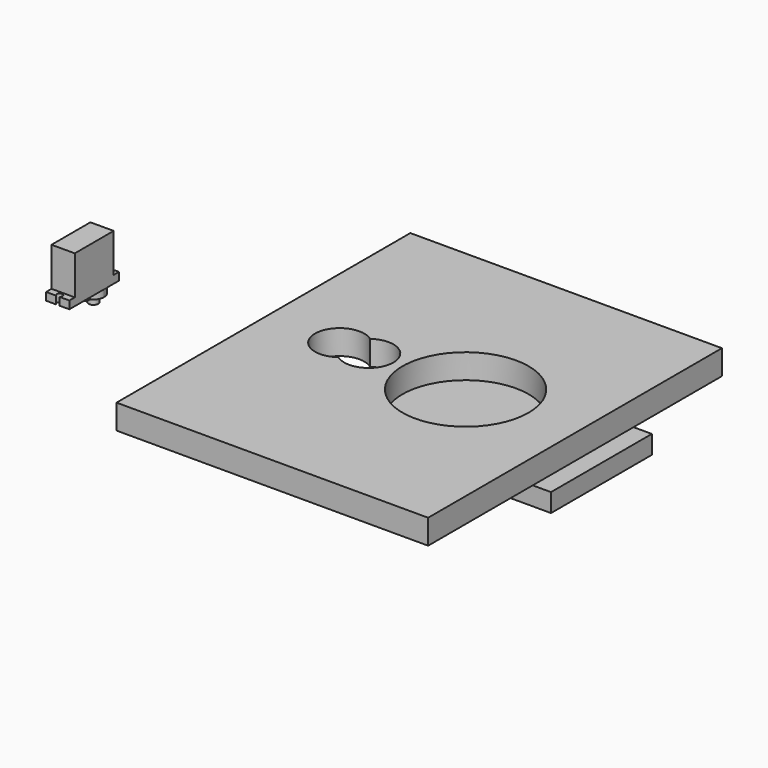
from build123d import *

# Parameters (mm, degrees)
F0_W      = 160.6854679329
F0_H      = 189.3717367202
F0_R      = 32.5
F1_DEPTH  = 12.7
F2_W      = 124
F2_H      = 65
F3_DEPTH  = 9.525
F5_DEPTH  = 12.7
F6_R      = 2.5
F7_DEPTH  = 24
F8_DEPTH  = 4
F9_DEPTH  = 8
F11_DEPTH = 20
F12_DEPTH = 4


# Not quite as in the source:
# - a length typed as a fraction of an inch, garbled in the dataset ("3 / 203.2 mm" for 3/8 in), is restored


with BuildPart() as f1:
    # F0 (on Top) → F1 (new body)
    with BuildSketch(Plane.XY):
        with Locations((-1.9587278366, 0.8332561702)):
            Rectangle(F0_W, F0_H)
        with Locations((20.2750398644, 2.9224749887)):
            Circle(F0_R, mode=Mode.SUBTRACT)
    extrude(amount=F1_DEPTH)

    # F4 (on face) → F5 (cut, through all)
    with BuildSketch(Plane.XY.offset(12.7)):
        with BuildLine():
            ThreePointArc((-37.3042601347, -7.1310623929), (-24.0579569753, -8.2077946527), (-17.1042601347, 3.1178399874))
            ThreePointArc((-17.1042601347, 3.1178399874), (-24.0579569753, 14.4434746274), (-37.3042601347, 13.3667423676))
            ThreePointArc((-37.3042601347, 13.3667423676), (-33.4786254946, 8.8641431468), (-32.1042601347, 3.1178399874))
            ThreePointArc((-32.1042601347, 3.1178399874), (-33.4786254946, -2.628463172), (-37.3042601347, -7.1310623929))
        make_face()
        with BuildLine():
            ThreePointArc((-32.1042601347, 3.1178399874), (-33.4786254946, 8.8641431468), (-37.3042601347, 13.3667423676))
            ThreePointArc((-37.3042601347, 13.3667423676), (-42.5042601347, 3.1178399874), (-37.3042601347, -7.1310623929))
            ThreePointArc((-37.3042601347, -7.1310623929), (-33.4786254946, -2.628463172), (-32.1042601347, 3.1178399874))
        make_face()
        with BuildLine():
            ThreePointArc((-37.3042601347, -7.1310623929), (-42.5042601347, 3.1178399874), (-37.3042601347, 13.3667423676))
            ThreePointArc((-37.3042601347, 13.3667423676), (-57.5042601347, 3.1178399874), (-37.3042601347, -7.1310623929))
        make_face()
    extrude(amount=-F5_DEPTH, mode=Mode.SUBTRACT)


with BuildPart() as f3:
    # F2 (on Top) → F3 (new body)
    with BuildSketch(Plane.XY):
        with Locations((25.8148865969, 6.0524680488)):
            Rectangle(F2_W, F2_H)
    extrude(amount=-F3_DEPTH)


with BuildPart() as f7:
    # F6 (on Top) → F7 (new body)
    with BuildSketch(Plane.XY):
        with BuildLine():
            Line((-170.091433923, 8.8584844804), (-175.1961884499, 8.8584844804))
            Line((-175.1961884499, 8.8584844804), (-175.1961884499, -23.1415155196))
            Line((-175.1961884499, -23.1415155196), (-170.091433923, -23.1415155196))
            ThreePointArc((-170.091433923, -23.1415155196), (-169.8696614598, -20.5976531011), (-167.6961884499, -21.9379642981))
            ThreePointArc((-167.6961884499, -21.9379642981), (-167.8558772528, -22.611437308), (-168.3009429767, -23.1415155196))
            Line((-168.3009429767, -23.1415155196), (-163.1961884499, -23.1415155196))
            Line((-163.1961884499, -23.1415155196), (-163.1961884499, 8.8584844804))
            Line((-163.1961884499, 8.8584844804), (-168.3009429767, 8.8584844804))
            ThreePointArc((-168.3009429767, 8.8584844804), (-167.8558772528, 8.3284062688), (-167.6961884499, 7.6549332589))
            ThreePointArc((-167.6961884499, 7.6549332589), (-169.8696614598, 6.3146220619), (-170.091433923, 8.8584844804))
        make_face()
        with BuildLine():
            ThreePointArc((-172.1793124567, -4.7622266293), (-171.827045531, 4.6884524947), (-163.6961884499, -0.1415155196))
            ThreePointArc((-163.6961884499, -0.1415155196), (-164.5558902937, -3.0940793244), (-166.8662368213, -5.1236160213))
            ThreePointArc((-166.8662368213, -5.1236160213), (-166.8311565651, -5.3751444183), (-166.8194298089, -5.6288364404))
            ThreePointArc((-166.8194298089, -5.6288364404), (-170.0083618757, -8.3435811136), (-172.1793124567, -4.7622266293))
        make_face(mode=Mode.SUBTRACT)
        with BuildLine():
            ThreePointArc((-168.3009429767, 8.8584844804), (-169.1961884499, 9.1549332589), (-170.091433923, 8.8584844804))
            Line((-170.091433923, 8.8584844804), (-168.3009429767, 8.8584844804))
        make_face()
        with BuildLine():
            Line((-168.3009429767, 8.8584844804), (-170.091433923, 8.8584844804))
            ThreePointArc((-170.091433923, 8.8584844804), (-169.8696614598, 6.3146220619), (-167.6961884499, 7.6549332589))
            ThreePointArc((-167.6961884499, 7.6549332589), (-167.8558772528, 8.3284062688), (-168.3009429767, 8.8584844804))
        make_face()
        with BuildLine():
            ThreePointArc((-167.6961884499, -21.9379642981), (-169.8696614598, -20.5976531011), (-170.091433923, -23.1415155196))
            Line((-170.091433923, -23.1415155196), (-168.3009429767, -23.1415155196))
            ThreePointArc((-168.3009429767, -23.1415155196), (-167.8558772528, -22.611437308), (-167.6961884499, -21.9379642981))
        make_face()
        with BuildLine():
            Line((-168.3009429767, -23.1415155196), (-170.091433923, -23.1415155196))
            ThreePointArc((-170.091433923, -23.1415155196), (-169.1961884499, -23.4379642981), (-168.3009429767, -23.1415155196))
        make_face()
        with BuildLine():
            ThreePointArc((-166.8662368213, -5.1236160213), (-164.5558902937, -3.0940793244), (-163.6961884499, -0.1415155196))
            ThreePointArc((-163.6961884499, -0.1415155196), (-171.827045531, 4.6884524947), (-172.1793124567, -4.7622266293))
            ThreePointArc((-172.1793124567, -4.7622266293), (-169.3828091294, -2.88517598), (-166.8662368213, -5.1236160213))
        make_face()
        with Locations((-169.1961884499, -0.1415155196)):
            Circle(F6_R, mode=Mode.SUBTRACT)
        with Locations((-169.1961884499, -0.1415155196)):
            Circle(F6_R)
        with BuildLine():
            ThreePointArc((-166.8662368213, -5.1236160213), (-169.5694298089, -5.6288364404), (-172.1793124567, -4.7622266293))
            ThreePointArc((-172.1793124567, -4.7622266293), (-170.0083618757, -8.3435811136), (-166.8194298089, -5.6288364404))
            ThreePointArc((-166.8194298089, -5.6288364404), (-166.8311565651, -5.3751444183), (-166.8662368213, -5.1236160213))
        make_face()
        with BuildLine():
            ThreePointArc((-166.8662368213, -5.1236160213), (-169.3828091294, -2.88517598), (-172.1793124567, -4.7622266293))
            ThreePointArc((-172.1793124567, -4.7622266293), (-169.5694298089, -5.6288364404), (-166.8662368213, -5.1236160213))
        make_face()
    extrude(amount=F7_DEPTH)

    # F6 (on Top) → F8 (join)
    with BuildSketch(Plane.XY):
        with BuildLine():
            ThreePointArc((-166.8662368213, -5.1236160213), (-164.5558902937, -3.0940793244), (-163.6961884499, -0.1415155196))
            ThreePointArc((-163.6961884499, -0.1415155196), (-171.827045531, 4.6884524947), (-172.1793124567, -4.7622266293))
            ThreePointArc((-172.1793124567, -4.7622266293), (-169.3828091294, -2.88517598), (-166.8662368213, -5.1236160213))
        make_face()
        with Locations((-169.1961884499, -0.1415155196)):
            Circle(F6_R, mode=Mode.SUBTRACT)
        with BuildLine():
            ThreePointArc((-166.8662368213, -5.1236160213), (-169.5694298089, -5.6288364404), (-172.1793124567, -4.7622266293))
            ThreePointArc((-172.1793124567, -4.7622266293), (-170.0083618757, -8.3435811136), (-166.8194298089, -5.6288364404))
            ThreePointArc((-166.8194298089, -5.6288364404), (-166.8311565651, -5.3751444183), (-166.8662368213, -5.1236160213))
        make_face()
        with BuildLine():
            ThreePointArc((-166.8662368213, -5.1236160213), (-169.3828091294, -2.88517598), (-172.1793124567, -4.7622266293))
            ThreePointArc((-172.1793124567, -4.7622266293), (-169.5694298089, -5.6288364404), (-166.8662368213, -5.1236160213))
        make_face()
    extrude(amount=-F8_DEPTH)

    # F6 (on Top) → F9 (join)
    with BuildSketch(Plane.XY):
        with Locations((-169.1961884499, -0.1415155196)):
            Circle(F6_R)
    extrude(amount=-F9_DEPTH)

    # F10 (on face) → F11 (cut)
    with BuildSketch(Plane.XY.offset(24)):
        with BuildLine():
            Line((-175.1961884499, 5.4334374145), (-163.1961884499, 5.4334374145))
            Line((-163.1961884499, 5.4334374145), (-163.1961884499, 8.8584844804))
            Line((-163.1961884499, 8.8584844804), (-168.3009429767, 8.8584844804))
            ThreePointArc((-168.3009429767, 8.8584844804), (-169.1961884499, 9.1549332589), (-170.091433923, 8.8584844804))
            Line((-170.091433923, 8.8584844804), (-175.1961884499, 8.8584844804))
            Line((-175.1961884499, 8.8584844804), (-175.1961884499, 5.4334374145))
        make_face()
        with BuildLine():
            Line((-163.1961884499, -23.1415155196), (-163.1961884499, -19.6447968483))
            Line((-163.1961884499, -19.6447968483), (-175.1961884499, -19.6447968483))
            Line((-175.1961884499, -19.6447968483), (-175.1961884499, -23.1415155196))
            Line((-175.1961884499, -23.1415155196), (-170.091433923, -23.1415155196))
            ThreePointArc((-170.091433923, -23.1415155196), (-169.1961884499, -23.4379642981), (-168.3009429767, -23.1415155196))
            Line((-168.3009429767, -23.1415155196), (-163.1961884499, -23.1415155196))
        make_face()
    extrude(amount=-F11_DEPTH, mode=Mode.SUBTRACT)

    # F6 (on Top) → F12 (cut, through all)
    with BuildSketch(Plane.XY):
        with BuildLine():
            Line((-168.3009429767, 8.8584844804), (-170.091433923, 8.8584844804))
            ThreePointArc((-170.091433923, 8.8584844804), (-169.8696614598, 6.3146220619), (-167.6961884499, 7.6549332589))
            ThreePointArc((-167.6961884499, 7.6549332589), (-167.8558772528, 8.3284062688), (-168.3009429767, 8.8584844804))
        make_face()
        with BuildLine():
            ThreePointArc((-167.6961884499, -21.9379642981), (-169.8696614598, -20.5976531011), (-170.091433923, -23.1415155196))
            Line((-170.091433923, -23.1415155196), (-168.3009429767, -23.1415155196))
            ThreePointArc((-168.3009429767, -23.1415155196), (-167.8558772528, -22.611437308), (-167.6961884499, -21.9379642981))
        make_face()
        with BuildLine():
            Line((-168.3009429767, -23.1415155196), (-170.091433923, -23.1415155196))
            ThreePointArc((-170.091433923, -23.1415155196), (-169.1961884499, -23.4379642981), (-168.3009429767, -23.1415155196))
        make_face()
        with BuildLine():
            ThreePointArc((-168.3009429767, 8.8584844804), (-169.1961884499, 9.1549332589), (-170.091433923, 8.8584844804))
            Line((-170.091433923, 8.8584844804), (-168.3009429767, 8.8584844804))
        make_face()
    extrude(amount=F12_DEPTH, mode=Mode.SUBTRACT)


solid = Compound([f1.part, f3.part, f7.part])
